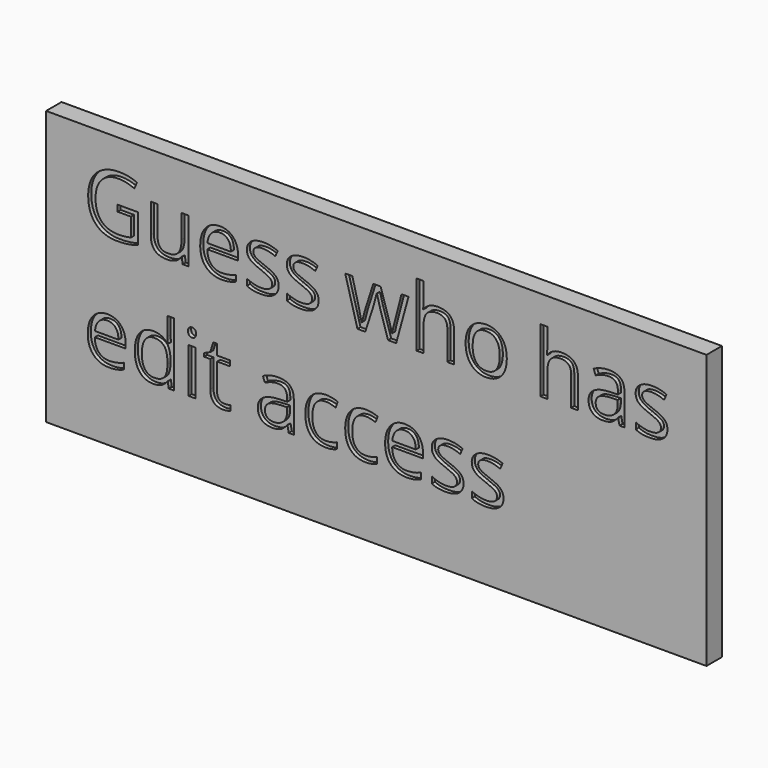
from build123d import *

# Parameters (mm, degrees)
F0_W         = 434.1324269772
F0_H         = 180.0699681044
F1_DEPTH     = 12.7
F2_TEXT_SIZE = 55.0940923858
F3_DEPTH     = 2.54


# Not quite as in the source:
# - Text() gives the source's letters only with a copy of the font that has no kerning and outlines rounded to 1/6400 em; it was checked with that copy


with BuildPart() as f1:
    # F0 (on Front) → F1 (new body)
    with BuildSketch(Plane.XZ):
        with Locations((217.0662134886, -90.0349840522)):
            Rectangle(F0_W, F0_H)
    extrude(amount=F1_DEPTH)

    # F2 (on face) → F3 (cut)
    with BuildSketch(Plane.XZ.offset(12.7)):
        with Locations((24.3085105903, -59.5618672669)):
            Text('Guess who has', F2_TEXT_SIZE, font='Open Sans', text_align=(TextAlign.LEFT, TextAlign.BOTTOM))
        with Locations((24.3085105903, -134.4898329116)):
            Text('edit access', F2_TEXT_SIZE, font='Open Sans', text_align=(TextAlign.LEFT, TextAlign.BOTTOM))
    extrude(amount=-F3_DEPTH, mode=Mode.SUBTRACT)


solid = f1.part
